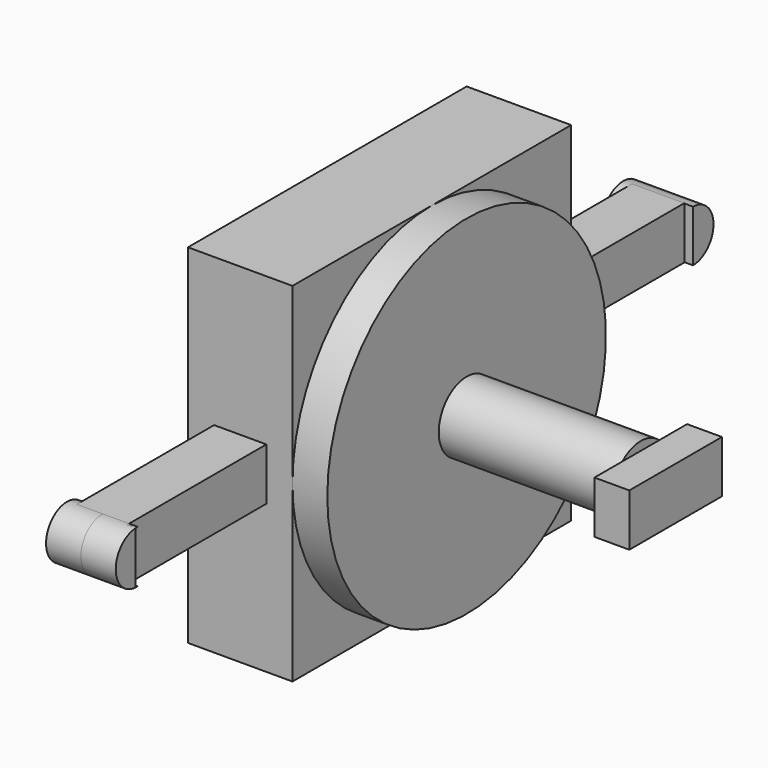
from build123d import *

# Parameters (mm, degrees)
F0_R      = 25.4
F1_DEPTH  = 127
F3_DEPTH  = 25.4
F4_DEPTH  = 25.4
F5_DEPTH  = 25.4
F6_R      = 127
F6_R_2    = 25.4
F7_DEPTH  = 25.4
F8_DEPTH  = 25.4
F9_R      = 25.4
F10_DEPTH = 76.2
F11_W     = 38.1
F11_H     = 38.1
F12_DEPTH = 127
F13_W     = 38.1
F13_H     = 38.1
F14_DEPTH = 127
F16_R     = 18.8423860879
F17_DEPTH = 25.4
F18_DEPTH = 25.4
F19_R     = 19.0757078593
F20_DEPTH = 25.4
F21_DEPTH = 25.4


with BuildPart() as f1:
    # F0 (on Right) → F1 (new body)
    with BuildSketch(Plane.YZ):
        Circle(F0_R)
    extrude(amount=F1_DEPTH)

    # F2 (on face) → F3 (join)
    with BuildSketch(Plane.YZ.offset(127)):
        Polygon((16.8005208253, 0), (0, 0), (-16.8005208253, 0), (-16.8005208253, -19.05), (16.8005208253, -19.05), align=None)
        Polygon((-16.8005208253, 0), (0, 0), (16.8005208253, 0), (16.8005208253, 19.05), (-16.8005208253, 19.05), align=None)
    extrude(amount=F3_DEPTH)

    # F4 (add): a face of the model
    f4_faces = [f1.faces().sort_by_distance(p)[0] for p in [
        (139.7, 16.8005208253, 0),
    ]]
    extrude(f4_faces, amount=F4_DEPTH)

    # F5 (add): a face of the model
    f5_faces = [f1.faces().sort_by_distance(p)[0] for p in [
        (139.7, -16.8005208253, 0),
    ]]
    extrude(f5_faces, amount=F5_DEPTH)


with BuildPart() as f7:
    # F6 (on face) → F7 (new body)
    with BuildSketch(Plane(origin=(0, 0, 0), x_dir=(0, -1, 0), z_dir=(-1, 0, 0))):
        Circle(F6_R)
        Circle(F6_R_2, mode=Mode.SUBTRACT)
    extrude(amount=F7_DEPTH)

    # F9 (on face) → F10 (join)
    with BuildSketch(Plane(origin=(-25.4, 0, 0), x_dir=(0, -1, 0), z_dir=(-1, 0, 0))):
        with BuildLine():
            Line((1.902e-07, -127), (127, -127))
            Line((127, -127), (127, 0))
            ThreePointArc((127, 0), (89.8025612779, -89.8025611435), (1.902e-07, -127))
        make_face()
        with BuildLine():
            Line((-127, -127), (1.902e-07, -127))
            ThreePointArc((1.902e-07, -127), (-89.8025611147, -89.8025613067), (-127, -8.12e-08))
            Line((-127, -8.12e-08), (-127, -127))
        make_face()
        with BuildLine():
            ThreePointArc((-127, -8.12e-08), (-89.8025611147, -89.8025613067), (1.902e-07, -127))
            ThreePointArc((1.902e-07, -127), (89.8025612779, -89.8025611435), (127, 0))
            ThreePointArc((127, 0), (89.8025611483, 89.802561273), (-1.763e-07, 127))
            ThreePointArc((-1.763e-07, 127), (-89.8025613018, 89.8025611196), (-127, -8.12e-08))
        make_face()
        Circle(F9_R, mode=Mode.SUBTRACT)
        with BuildLine():
            ThreePointArc((-1.763e-07, 127), (89.8025611483, 89.802561273), (127, 0))
            Line((127, 0), (127, 127))
            Line((127, 127), (-1.763e-07, 127))
        make_face()
        with BuildLine():
            Line((-127, 127), (-127, -8.12e-08))
            ThreePointArc((-127, -8.12e-08), (-89.8025613018, 89.8025611196), (-1.763e-07, 127))
            Line((-1.763e-07, 127), (-127, 127))
        make_face()
    extrude(amount=F10_DEPTH)

    # F11 (on face) → F12 (join)
    with BuildSketch(Plane(origin=(0, 127, 0), x_dir=(-1, 0, 0), z_dir=(0, 1, 0))):
        with Locations((63.5, 0)):
            Rectangle(F11_W, F11_H)
    extrude(amount=F12_DEPTH)

    # F13 (on face) → F14 (join)
    with BuildSketch(Plane.XZ.offset(127)):
        with Locations((-63.5, 0)):
            Rectangle(F13_W, F13_H)
    extrude(amount=F14_DEPTH)

    # F16 (on offset) → F17 (join)
    with BuildSketch(Plane(origin=(-63.5, 0, 0), x_dir=(0, -1, 0), z_dir=(-1, 0, 0))):
        with Locations((-253.818333149, 0)):
            Circle(F16_R)
    extrude(amount=F17_DEPTH)

    # F18 (add): a face of the model
    f18_faces = [f7.faces().sort_by_distance(p)[0] for p in [
        (-63.5, 261.9135488833, 0),
    ]]
    extrude(f18_faces, amount=F18_DEPTH)

    # F19 (on offset) → F20 (join)
    with BuildSketch(Plane(origin=(-63.5, 0, 0), x_dir=(0, -1, 0), z_dir=(-1, 0, 0))):
        with Locations((253.1379759312, 0)):
            Circle(F19_R)
    extrude(amount=F20_DEPTH)

    # F21 (add): a face of the model
    f21_faces = [f7.faces().sort_by_distance(p)[0] for p in [
        (-63.5, -261.7006711899, 0),
    ]]
    extrude(f21_faces, amount=F21_DEPTH)


with BuildPart() as f8:
    # F8 (new): a face of the model
    f8_faces = [f1.part.faces().sort_by_distance(p)[0] for p in [
        (0, 0, 0),
    ]]
    extrude(f8_faces, amount=F8_DEPTH)


solid = Compound([f1.part, f7.part, f8.part])
